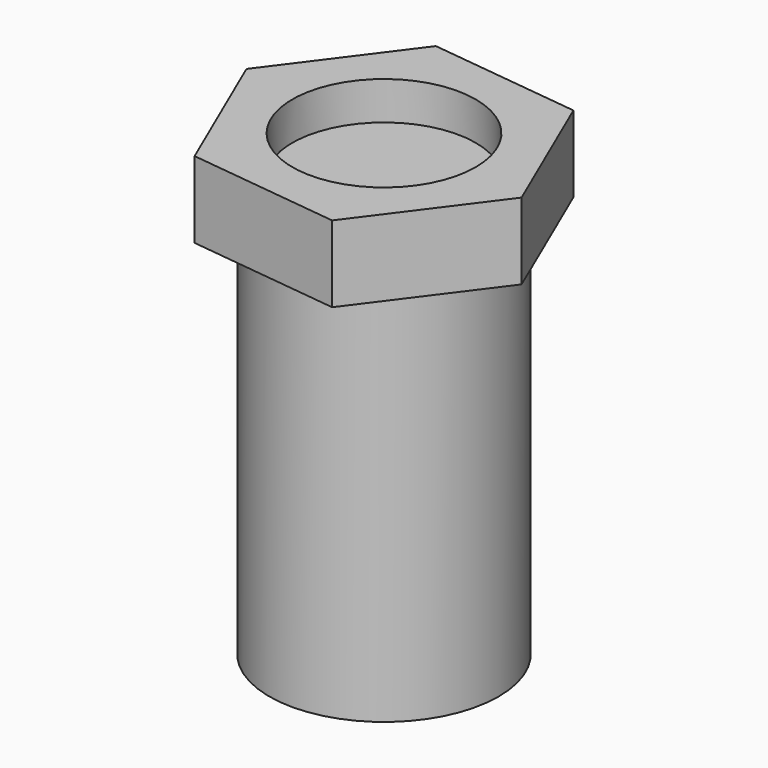
from build123d import *

# Parameters (mm, degrees)
F0_W     = 0.75
F0_H     = 2.5
F2_R     = 0.75
F3_DEPTH = 0.5
F4_R     = 0.6
F5_DEPTH = 0.25


with BuildPart() as f1:
    # F0 (on Front) → F1 (revolve)
    with BuildSketch(Plane.XZ):
        with Locations((-0.375, 1.25)):
            Rectangle(F0_W, F0_H)
    revolve(axis=Axis((0, 0, 1.25), (0, 0, 1)))

    # F2 (on face) → F3 (join)
    with BuildSketch(Plane.XY.offset(2.5)):
        Polygon((0.5977295956, 0.80169778), (-0.3954258459, 0.9184979044), (-0.9931554415, 0.1168001244), (-0.5977295956, -0.80169778), (0.3954258459, -0.9184979044), (0.9931554415, -0.1168001244), align=None)
        Circle(F2_R, mode=Mode.SUBTRACT)
        Circle(F2_R)
    extrude(amount=F3_DEPTH)

    # F4 (on face) → F5 (cut)
    with BuildSketch(Plane.XY.offset(3)):
        Circle(F4_R)
    extrude(amount=-F5_DEPTH, mode=Mode.SUBTRACT)


solid = f1.part
